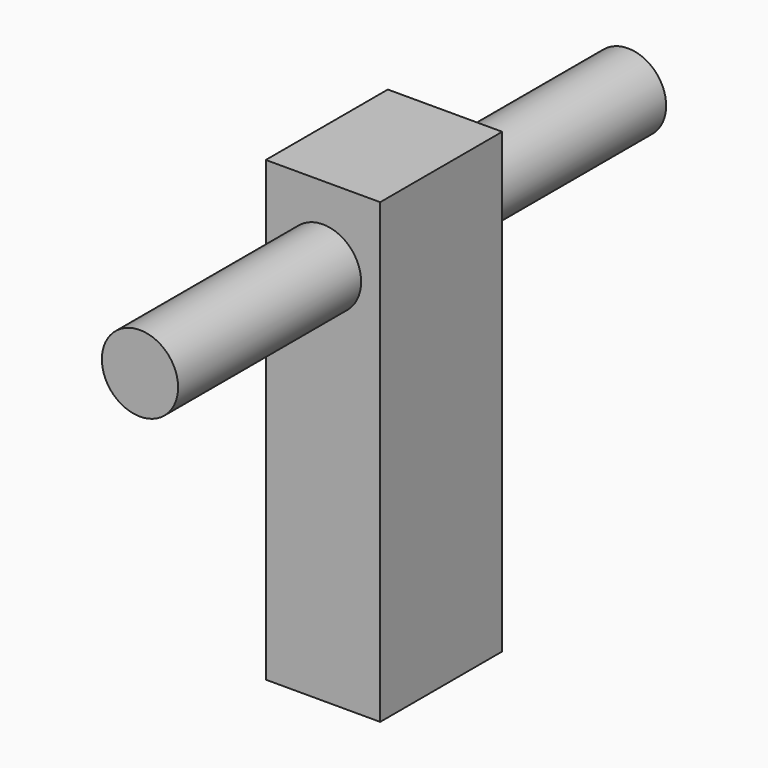
from build123d import *

# Parameters (mm, degrees)
F0_W     = 9.525
F0_H     = 38.1
F0_R     = 2.38125
F1_DEPTH = 12.7
F2_R     = 2.38125
F3_DEPTH = 12.7
F2_R_2   = 3.175
F4_DEPTH = 19.05
F5_R     = 3.175
F5_R_2   = 2.38125
F6_DEPTH = 19.05


with BuildPart() as f1:
    # F0 (on Front) → F1 (new body)
    with BuildSketch(Plane.XZ):
        Rectangle(F0_W, F0_H)
        with Locations((0, 12.7)):
            Circle(F0_R, mode=Mode.SUBTRACT)
    extrude(amount=F1_DEPTH)


with BuildPart() as f3:
    # F2 (on face) → F3 (new body)
    with BuildSketch(Plane.XZ.offset(12.7)):
        with Locations((0, 12.7)):
            Circle(F2_R)
    extrude(amount=-F3_DEPTH)

    # F2 (on face) → F4 (join)
    with BuildSketch(Plane.XZ.offset(12.7)):
        with Locations((0, 12.7)):
            Circle(F2_R_2)
        with Locations((0, 12.7)):
            Circle(F2_R, mode=Mode.SUBTRACT)
        with Locations((0, 12.7)):
            Circle(F2_R)
    extrude(amount=F4_DEPTH)

    # F5 (on face) → F6 (join)
    with BuildSketch(Plane(origin=(0, 0, 0), x_dir=(-1, 0, 0), z_dir=(0, 1, 0))):
        with Locations((0, 12.7)):
            Circle(F5_R)
        with Locations((0, 12.7)):
            Circle(F5_R_2, mode=Mode.SUBTRACT)
        with Locations((0, 12.7)):
            Circle(F5_R_2)
    extrude(amount=F6_DEPTH)


solid = Compound([f1.part, f3.part])
